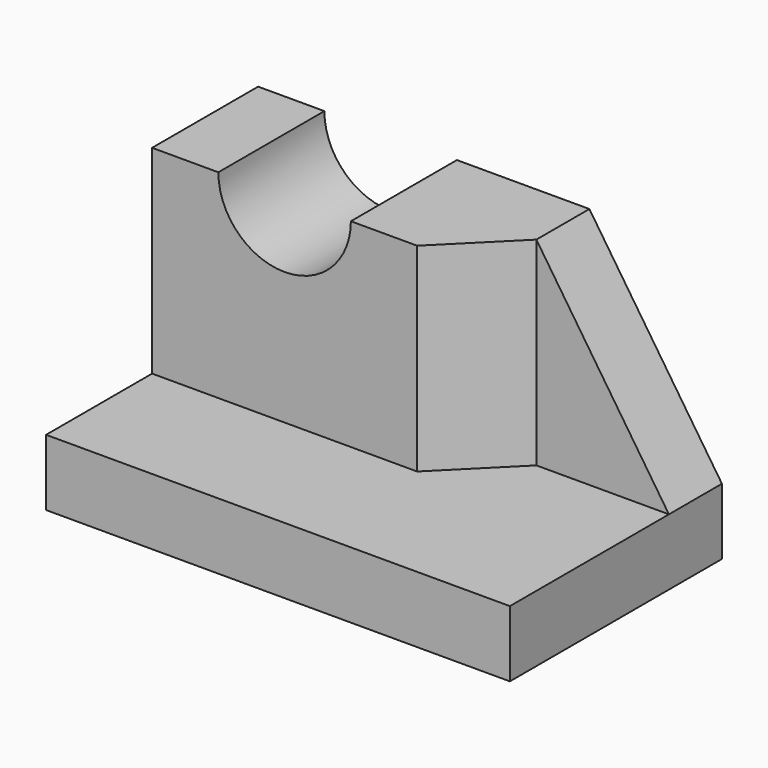
from build123d import *

# Parameters (mm, degrees)
F0_W     = 254
F0_H     = 762
F1_DEPTH = 1016
F2_R     = 254
F3_DEPTH = 1064.26
F5_DEPTH = 508
F7_DEPTH = 254
F9_DEPTH = 762


with BuildPart() as f1:
    # F0 (on Front) → F1 (new body)
    with BuildSketch(Plane.XZ):
        with BuildLine():
            Line((0, 1016), (0, 254))
            Line((0, 254), (1016, 254))
            Line((1016, 254), (1016, 1016))
            Line((1016, 1016), (762, 1016))
            ThreePointArc((762, 1016), (508, 762), (254, 1016))
            Line((254, 1016), (0, 1016))
        make_face()
        Polygon((0, 254), (0, 0), (1778, 0), (1778, 254), (1270, 254), (1016, 254), align=None)
        with Locations((1143, 635)):
            Rectangle(F0_W, F0_H)
        Polygon((1270, 254), (1778, 254), (1270, 1016), align=None)
    extrude(amount=F1_DEPTH)

    # F2 (on face) → F3 (cut)
    with BuildSketch(Plane.XZ.offset(1016)):
        with Locations((508, 1016)):
            Circle(F2_R)
    extrude(amount=-F3_DEPTH, mode=Mode.SUBTRACT)

    # F4 (on face) → F5 (cut)
    with BuildSketch(Plane.XZ.offset(1016)):
        Polygon((1270, 254), (1270, 1016), (254, 1016), (0, 1016), (0, 254), align=None)
        Polygon((1778, 254), (1270, 1016), (1270, 254), align=None)
    extrude(amount=-F5_DEPTH, mode=Mode.SUBTRACT)

    # F6 (on face) → F7 (cut)
    with BuildSketch(Plane.XZ.offset(508)):
        Polygon((1778, 254), (1270, 1016), (1270, 254), align=None)
    extrude(amount=-F7_DEPTH, mode=Mode.SUBTRACT)

    # F8 (on face) → F9 (cut)
    with BuildSketch(Plane.XY.offset(1016)):
        Polygon((1270, -508), (1270, -254), (1016, -508), align=None)
    extrude(amount=-F9_DEPTH, mode=Mode.SUBTRACT)


solid = f1.part
